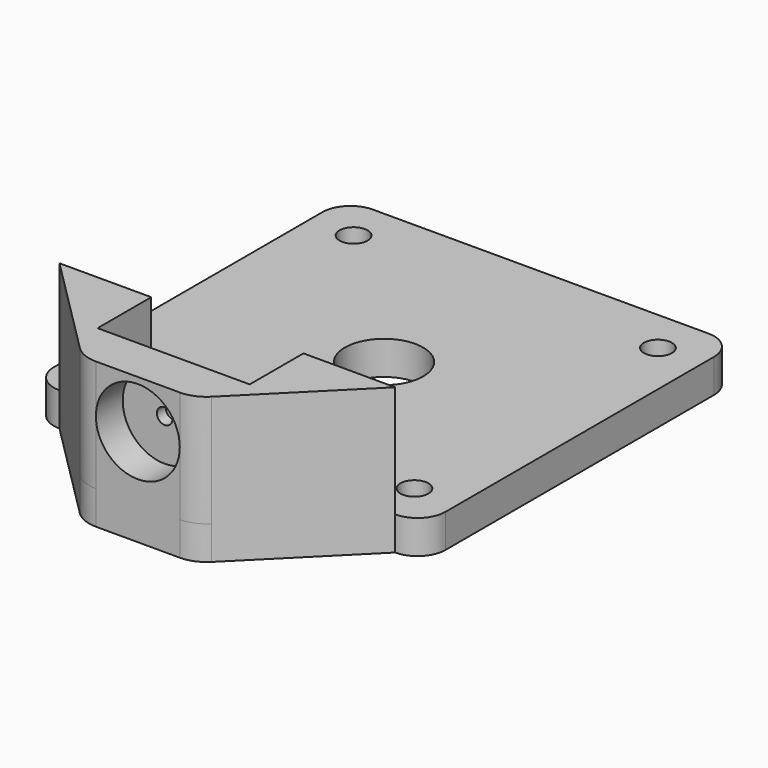
from build123d import *

# Parameters (mm, degrees)
F0_W        = 20.32
F0_H        = 50.8
F1_DEPTH    = 7.62
F2_D        = 6.35
F3_R        = 6.35
F4_D        = 17.78
F5_DEPTH    = 25.4
F6_T1_DEPTH = 138.2614957887
F7_R        = 7.62
F9_DEPTH    = 25.4
F11_D       = 4.318
F11_DEPTH   = 5.08
F11_TIP     = 1.2972580765
F12_D       = 3.556
F13_R       = 9.525
F13_R_2     = 1.778
F14_DEPTH   = 7.62
F10_W       = 5.588
F10_H       = 25.4
F16_DEPTH   = 15.24
F17_DEPTH   = 25.4


# Not quite as in the source:
# - a fillet or chamfer that OpenCascade refuses, or shapes differently, is made with other operations: its cross-section is extruded or revolved along the edge and cut away or added


with BuildPart() as f1:
    # F0 (on Top) → F1 (new body)
    with BuildSketch(Plane.XY):
        Polygon((46.4461110532, 37.6075126914), (-42.4538889468, 37.6075126914), (-42.4538889468, -51.2924873086), (46.4461110532, -51.2924873086), (46.4461110532, -32.2424873086), (26.1261110532, -32.2424873086), (26.1261110532, 18.5575126914), (46.4461110532, 18.5575126914), align=None)
        with Locations((36.2861110532, -6.8424873086)):
            Rectangle(F0_W, F0_H)
    extrude(amount=F1_DEPTH)

    # F2 (through all)
    with Locations(Plane(origin=(0, 0, 0), x_dir=(1, 0, 0), z_dir=(0, 0, -1))):
        with Locations((-32.5478889468, -27.7015126914), (36.5401110532, -27.7015126914), (36.5401110532, 41.3864873086), (-32.5478889468, 41.3864873086)):
            Hole(F2_D / 2)

    # F3
    f3_edges = [f1.edges().sort_by_distance(p)[0] for p in [
        (-42.453889, -51.292487, 3.81),
        (46.446111, -51.292487, 3.81),
        (46.446111, 37.607513, 3.81),
        (-42.453889, 37.607513, 3.81),
    ]]
    fillet(f3_edges, radius=F3_R)

    # F4 (through all)
    with Locations(Plane(origin=(0, 0, 0), x_dir=(1, 0, 0), z_dir=(0, 0, -1))):
        with Locations((1.9961110532, 6.8424873086)):
            Hole(F4_D / 2)

    # F5 (add): a face of the model
    f5_faces = [f1.faces().sort_by_distance(p)[0] for p in [
        (1.9961110532, -51.2924873086, 3.81),
    ]]
    extrude(f5_faces, amount=F5_DEPTH)

    # F6: chamfer of 25.4 on 3 edges, made by hand

    # F6_s2 → F6_t1 (cut)
    with BuildSketch(Plane.XY.offset(-65.3207478943)):
        Polygon((40.0961110532, -51.2924873086), (14.6961110532, -76.6924873086), (40.0961110532, -76.6924873086), align=None)
        Polygon((-36.1038889468, -51.2924873086), (-10.7038889468, -76.6924873086), (-36.1038889468, -76.6924873086), align=None)
    extrude(amount=F6_T1_DEPTH, mode=Mode.SUBTRACT)

    # F7
    f7_edges = [f1.edges().sort_by_distance(p)[0] for p in [
        (14.696111, -76.692487, 3.81),
        (-10.703889, -76.692487, 3.81),
    ]]
    fillet(f7_edges, radius=F7_R)

    # F8 (on face) → F9 (join)
    with BuildSketch(Plane.XY.offset(7.62)):
        with BuildLine():
            Line((24.8561110532, -66.5324873086), (-20.8638889468, -66.5324873086))
            Line((-20.8638889468, -66.5324873086), (-12.9357352742, -74.4606409812))
            ThreePointArc((-12.9357352742, -74.4606409812), (-10.4636293562, -76.1124493463), (-7.5475816015, -76.6924873086))
            Line((-7.5475816015, -76.6924873086), (11.5398037079, -76.6924873086))
            ThreePointArc((11.5398037079, -76.6924873086), (14.4558514626, -76.1124493463), (16.9279573806, -74.4606409812))
            Line((16.9279573806, -74.4606409812), (24.8561110532, -66.5324873086))
        make_face()
    extrude(amount=F9_DEPTH)

    # F11
    with Locations(Plane(origin=(0, -66.5324873086, 0), x_dir=(-1, 0, 0), z_dir=(0, 1, 0))):
        with Locations((-14.6961110532, 22.098), (10.7038889468, 22.098)):
            Hole(F11_D / 2, depth=F11_DEPTH)
            with Locations((0, 0, -(F11_DEPTH + F11_TIP / 2))):  # 118° drill point
                Cone(0, F11_D / 2, F11_TIP, mode=Mode.SUBTRACT)

    # F12 (through all)
    with Locations(Plane(origin=(0, -66.5324873086, 0), x_dir=(-1, 0, 0), z_dir=(0, 1, 0))):
        with Locations((-1.9961110532, 22.098)):
            Hole(F12_D / 2)

    # F13 (on face) → F14 (cut)
    with BuildSketch(Plane.XZ.offset(76.6924873086)):
        with Locations((1.9961110532, 22.098)):
            Circle(F13_R)
        with Locations((1.9961110532, 22.098)):
            Circle(F13_R_2, mode=Mode.SUBTRACT)
    extrude(amount=-F14_DEPTH, mode=Mode.SUBTRACT)

    # F10 (on face) → F16 (join)
    with BuildSketch(Plane(origin=(0, -66.5324873086, 0), x_dir=(-1, 0, 0), z_dir=(0, 1, 0))):
        with Locations((-22.0621110532, 20.32)):
            Rectangle(F10_W, F10_H)
        with Locations((18.0698889468, 20.32)):
            Rectangle(F10_W, F10_H)
    extrude(amount=F16_DEPTH)

    # F15 (on face) → F17 (join)
    with BuildSketch(Plane.XY.offset(7.62)):
        Polygon((24.8561110532, -66.5324873086), (40.0961110532, -51.2924873086), (24.8561110532, -51.2924873086), align=None)
        Polygon((-36.1038889468, -51.2924873086), (-20.8638889468, -66.5324873086), (-20.8638889468, -51.2924873086), align=None)
    extrude(amount=F17_DEPTH)


solid = f1.part
